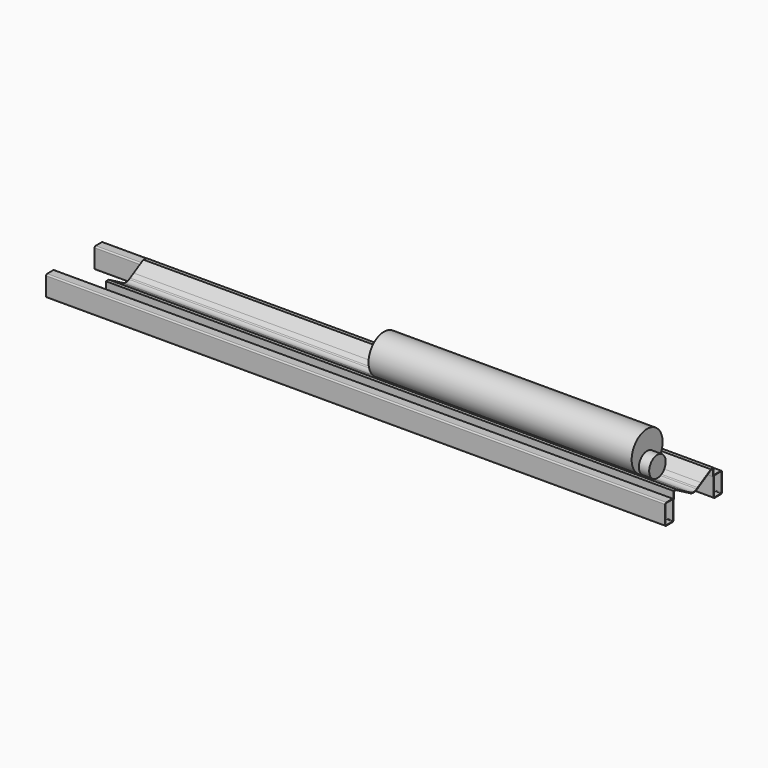
from build123d import *

# Parameters (mm, degrees)
F1_DEPTH = 6096
F2_DEPTH = 5588
F3_START = -355.6
F3_DEPTH = 2692.4
F4_START = -457.2
F4_DEPTH = 2590.8


# Not quite as in the source:
# - a feature names something its author has since deleted; it is built from what else it names


with BuildPart() as f1:
    # F0 (on Right) → F1 (new body)
    with BuildSketch(Plane.YZ):
        with BuildLine():
            Line((-278.751844046, 57.15), (-336.55, 57.15))
            ThreePointArc((-336.55, 57.15), (-345.5302561211, 53.4302561211), (-349.25, 44.45))
            Line((-349.25, 44.45), (-349.25, -133.35))
            ThreePointArc((-349.25, -133.35), (-345.5302561211, -142.3302561211), (-336.55, -146.05))
            Line((-336.55, -146.05), (-260.35, -146.05))
            ThreePointArc((-260.35, -146.05), (-251.3697438789, -142.3302561211), (-247.65, -133.35))
            Line((-247.65, -133.35), (-247.65, 44.45))
            ThreePointArc((-247.65, 44.45), (-251.3697438789, 53.4302561211), (-260.35, 57.15))
            Line((-260.35, 57.15), (-268.1402802436, 57.15))
            Line((-268.1402802436, 57.15), (-269.3472818438, 57.15))
            Line((-269.3472818438, 57.15), (-278.751844046, 57.15))
        make_face()
        with BuildLine():
            ThreePointArc((-342.9, 44.45), (-341.0401280605, 48.9401280605), (-336.55, 50.8))
            Line((-336.55, 50.8), (-260.35, 50.8))
            ThreePointArc((-260.35, 50.8), (-255.8598719395, 48.9401280605), (-254, 44.45))
            Line((-254, 44.45), (-254, -133.35))
            ThreePointArc((-254, -133.35), (-255.8598719395, -137.8401280605), (-260.35, -139.7))
            Line((-260.35, -139.7), (-336.55, -139.7))
            ThreePointArc((-336.55, -139.7), (-341.0401280605, -137.8401280605), (-342.9, -133.35))
            Line((-342.9, -133.35), (-342.9, 44.45))
        make_face(mode=Mode.SUBTRACT)
    extrude(amount=-F1_DEPTH)


with BuildPart() as f1b:
    # F0 (on Right) → F1, piece 2 (new body)
    with BuildSketch(Plane.YZ):
        with BuildLine():
            ThreePointArc((260.35, 57.15), (251.3697438789, 53.4302561211), (247.65, 44.45))
            Line((247.65, 44.45), (247.65, -133.35))
            ThreePointArc((247.65, -133.35), (251.3697438789, -142.3302561211), (260.35, -146.05))
            Line((260.35, -146.05), (336.55, -146.05))
            ThreePointArc((336.55, -146.05), (345.5302561211, -142.3302561211), (349.25, -133.35))
            Line((349.25, -133.35), (349.25, 44.45))
            ThreePointArc((349.25, 44.45), (345.5302561211, 53.4302561211), (336.55, 57.15))
            Line((336.55, 57.15), (260.35, 57.15))
        make_face()
        with BuildLine():
            Line((260.35, 50.8), (336.55, 50.8))
            ThreePointArc((336.55, 50.8), (341.0401280605, 48.9401280605), (342.9, 44.45))
            Line((342.9, 44.45), (342.9, -133.35))
            ThreePointArc((342.9, -133.35), (341.0401280605, -137.8401280605), (336.55, -139.7))
            Line((336.55, -139.7), (260.35, -139.7))
            ThreePointArc((260.35, -139.7), (255.8598719395, -137.8401280605), (254, -133.35))
            Line((254, -133.35), (254, 44.45))
            ThreePointArc((254, 44.45), (255.8598719395, 48.9401280605), (260.35, 50.8))
        make_face(mode=Mode.SUBTRACT)
    extrude(amount=-F1_DEPTH)


with BuildPart() as f2:
    # F0 (on Right) → F2 (new body)
    with BuildSketch(Plane.YZ):
        with BuildLine():
            Line((-247.65, 120.65), (-247.65, 44.45))
            Line((-247.65, 44.45), (-241.3, 44.45))
            Line((-241.3, 44.45), (-241.3, 114.3))
            Line((-241.3, 114.3), (-214.7923633436, 114.3))
            Line((-214.7923633436, 114.3), (-40.6681247176, 15.7258547021))
            ThreePointArc((-40.6681247176, 15.7258547021), (0, 5.0132135897), (40.6681247176, 15.7258547021))
            Line((40.6681247176, 15.7258547021), (214.7923633436, 114.3))
            Line((214.7923633436, 114.3), (241.3, 114.3))
            Line((241.3, 114.3), (241.3, 44.45))
            Line((241.3, 44.45), (247.65, 44.45))
            Line((247.65, 44.45), (247.65, 120.65))
            Line((247.65, 120.65), (213.1196707487, 120.65))
            Line((213.1196707487, 120.65), (93.8495232493, 53.1295161083))
            Line((93.8495232493, 53.1295161083), (50.0530768875, 28.3357406909))
            Line((50.0530768875, 28.3357406909), (37.5398074317, 21.2518053858))
            ThreePointArc((37.5398074317, 21.2518053858), (0, 11.3632135897), (-37.5398074317, 21.2518053858))
            Line((-37.5398074317, 21.2518053858), (-50.0530764944, 28.3357404684))
            Line((-50.0530764944, 28.3357404684), (-93.8495233688, 53.1295161759))
            Line((-93.8495233688, 53.1295161759), (-213.1196707487, 120.65))
            Line((-213.1196707487, 120.65), (-247.65, 120.65))
        make_face()
    extrude(amount=-F2_DEPTH)


with BuildPart() as f3:
    # F0 (on Right) → F3 (new body)
    with BuildSketch(Plane.YZ.offset(F3_START)):
        with BuildLine():
            ThreePointArc((-67.4075244001, 40.7326269894), (-59.0564889701, 34.0775511932), (-50.0530764944, 28.3357404684))
            ThreePointArc((-50.0530764944, 28.3357404684), (2.258e-07, 15.150951453), (50.0530768875, 28.3357406909))
            ThreePointArc((50.0530768875, 28.3357406909), (59.0564891539, 34.0775513244), (67.4075244001, 40.7326269894))
            ThreePointArc((67.4075244001, 40.7326269894), (0, 28.4080339743), (-67.4075244001, 40.7326269894))
        make_face()
        with BuildLine():
            ThreePointArc((101.6, 116.750951453), (-41.6770651615, 209.4093684453), (-67.4075244001, 40.7326269894))
            ThreePointArc((-67.4075244001, 40.7326269894), (0, 28.4080339743), (67.4075244001, 40.7326269894))
            ThreePointArc((67.4075244001, 40.7326269894), (92.6584169923, 75.0738862915), (101.6, 116.750951453))
        make_face()
    extrude(amount=-F3_DEPTH)


with BuildPart() as f4:
    # F0 (on Right) → F4 (new body)
    with BuildSketch(Plane.YZ.offset(F4_START)):
        with BuildLine():
            ThreePointArc((190.5, 218.9080339743), (-95.9476831358, 383.4810940446), (-93.8495233688, 53.1295161759))
            ThreePointArc((-93.8495233688, 53.1295161759), (-80.8664304836, 46.4236276622), (-67.4075244001, 40.7326269894))
            ThreePointArc((-67.4075244001, 40.7326269894), (-41.6770651615, 209.4093684453), (101.6, 116.750951453))
            ThreePointArc((101.6, 116.750951453), (92.6584169923, 75.0738862915), (67.4075244001, 40.7326269894))
            ThreePointArc((67.4075244001, 40.7326269894), (80.8664304214, 46.4236276331), (93.8495232493, 53.1295161083))
            ThreePointArc((93.8495232493, 53.1295161083), (164.5730600356, 122.9603507793), (190.5, 218.9080339743))
        make_face()
        with BuildLine():
            ThreePointArc((101.6, 116.750951453), (-41.6770651615, 209.4093684453), (-67.4075244001, 40.7326269894))
            ThreePointArc((-67.4075244001, 40.7326269894), (0, 28.4080339743), (67.4075244001, 40.7326269894))
            ThreePointArc((67.4075244001, 40.7326269894), (92.6584169923, 75.0738862915), (101.6, 116.750951453))
        make_face()
    extrude(amount=-F4_DEPTH)


solid = Compound([f1.part, f1b.part, f2.part, f3.part, f4.part])
